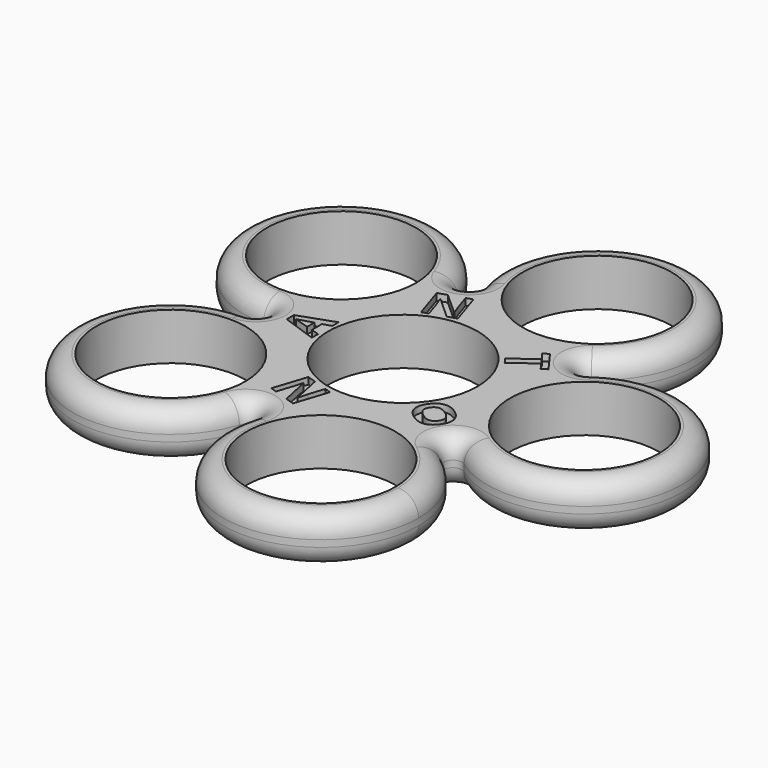
from build123d import *

# Parameters (mm, degrees)
F1_R         = 11.1
F2_DEPTH     = 3.5
F3_R         = 3
F4_TEXT_SIZE = 7.2184329232
F5_DEPTH     = 1


# Not quite as in the source:
# - Text() gives the source's letters only with a copy of the font that has no kerning and outlines rounded to 1/6400 em; it was checked with that copy


with BuildPart() as f2:
    # F1 (on Top) → F2 (new body, symmetric)
    with BuildSketch(Plane.XY):
        with BuildLine():
            ThreePointArc((18.4771138418, -11.7307464184), (33.5828622462, -12.9195946007), (41.5, 0))
            ThreePointArc((41.5, 0), (33.5828622462, 12.9195946007), (18.4771138418, 11.7307464184))
            ThreePointArc((18.4771138418, 11.7307464184), (12.5, 0), (18.4771138418, -11.7307464184))
        make_face()
        with Locations((27, 0)):
            Circle(F1_R, mode=Mode.SUBTRACT)
        with BuildLine():
            ThreePointArc((18.4771138418, -11.7307464184), (12.5, 0), (18.4771138418, 11.7307464184))
            ThreePointArc((18.4771138418, 11.7307464184), (16.5632128725, 12.0338785523), (16.8663450064, 13.9477795215))
            ThreePointArc((16.8663450064, 13.9477795215), (3.8627124297, 11.8882064537), (-5.4468606382, 21.1977795215))
            ThreePointArc((-5.4468606382, 21.1977795215), (-6.3265843544, 19.4712245141), (-8.0531393618, 20.3509482303))
            ThreePointArc((-8.0531393618, 20.3509482303), (-7.5219779095, 18.138501555), (-7.3434588481, 15.8702018119))
            ThreePointArc((-7.3434588481, 15.8702018119), (-11.5904105209, 5.6171534847), (-21.8434588481, 1.3702018119))
            ThreePointArc((-21.8434588481, 1.3702018119), (-20.4732570362, 0), (-21.8434588481, -1.3702018119))
            ThreePointArc((-21.8434588481, -1.3702018119), (-11.5904105209, -5.6171534847), (-7.3434588481, -15.8702018119))
            ThreePointArc((-7.3434588481, -15.8702018119), (-7.5219779095, -18.138501555), (-8.0531393618, -20.3509482303))
            ThreePointArc((-8.0531393618, -20.3509482303), (-6.3265843544, -19.4712245141), (-5.4468606382, -21.1977795215))
            ThreePointArc((-5.4468606382, -21.1977795215), (3.8627124297, -11.8882064537), (16.8663450064, -13.9477795215))
            ThreePointArc((16.8663450064, -13.9477795215), (16.5632128725, -12.0338785523), (18.4771138418, -11.7307464184))
        make_face()
        Circle(F1_R, mode=Mode.SUBTRACT)
        with BuildLine():
            ThreePointArc((-5.4468606382, 21.1977795215), (3.8627124297, 11.8882064537), (16.8663450064, 13.9477795215))
            ThreePointArc((16.8663450064, 13.9477795215), (21.2630534489, 19.0956636937), (22.8434588481, 25.67852594))
            ThreePointArc((22.8434588481, 25.67852594), (6.075159105, 40.0000068786), (-5.4468606382, 21.1977795215))
        make_face()
        with Locations((8.3434588481, 25.67852594)):
            Circle(F1_R, mode=Mode.SUBTRACT)
        with BuildLine():
            ThreePointArc((22.8434588481, -25.67852594), (21.2630534489, -19.0956636937), (16.8663450064, -13.9477795215))
            ThreePointArc((16.8663450064, -13.9477795215), (3.8627124297, -11.8882064537), (-5.4468606382, -21.1977795215))
            ThreePointArc((-5.4468606382, -21.1977795215), (6.075159105, -40.0000068786), (22.8434588481, -25.67852594))
        make_face()
        with Locations((8.3434588481, -25.67852594)):
            Circle(F1_R, mode=Mode.SUBTRACT)
        with BuildLine():
            ThreePointArc((-7.3434588481, 15.8702018119), (-7.5219779095, 18.138501555), (-8.0531393618, 20.3509482303))
            ThreePointArc((-8.0531393618, 20.3509482303), (-33.5742052666, 24.3930879701), (-21.8434588481, 1.3702018119))
            ThreePointArc((-21.8434588481, 1.3702018119), (-11.5904105209, 5.6171534847), (-7.3434588481, 15.8702018119))
        make_face()
        with Locations((-21.8434588481, 15.8702018119)):
            Circle(F1_R, mode=Mode.SUBTRACT)
        with BuildLine():
            ThreePointArc((-21.8434588481, -1.3702018119), (-33.5742052666, -24.3930879701), (-8.0531393618, -20.3509482303))
            ThreePointArc((-8.0531393618, -20.3509482303), (-7.5219779095, -18.138501555), (-7.3434588481, -15.8702018119))
            ThreePointArc((-7.3434588481, -15.8702018119), (-11.5904105209, -5.6171534847), (-21.8434588481, -1.3702018119))
        make_face()
        with Locations((-21.8434588481, -15.8702018119)):
            Circle(F1_R, mode=Mode.SUBTRACT)
    extrude(amount=F2_DEPTH, both=True)

    # F3
    f3_edges = [f2.edges().sort_by_distance(p)[0] for p in [
        (-33.574205, -24.393088, 3.5),
        (-33.574205, -24.393088, -3.5),
    ]]
    fillet(f3_edges, radius=F3_R)

    # F4 (on face) → F5 (cut, symmetric)
    with BuildSketch(Plane.XY.offset(3.5)):
        with Locations(Location((-11.5846967189, -2.4733702824), (0, 0, 90))):
            Text('A', F4_TEXT_SIZE, font='Open Sans', font_style=FontStyle.BOLD, text_align=(TextAlign.LEFT, TextAlign.BOTTOM))
        with Locations(Location((-6.3101283431, 10.2808768785), (0, 0, 18))):
            Text('N', F4_TEXT_SIZE, font='Open Sans', font_style=FontStyle.BOLD, text_align=(TextAlign.LEFT, TextAlign.BOTTOM))
        with Locations(Location((8.2989238401, 8.7424773108), (0, 0, -54))):
            Text('T', F4_TEXT_SIZE, font='Open Sans', font_style=FontStyle.BOLD, text_align=(TextAlign.LEFT, TextAlign.BOTTOM))
        with Locations(Location((11.122600367, -4.7498141065), (0, 0, -126))):
            Text('O', F4_TEXT_SIZE, font='Open Sans', font_style=FontStyle.BOLD, text_align=(TextAlign.LEFT, TextAlign.BOTTOM))
        with Locations(Location((-0.7597079111, -12.0412665495), (0, 0, 162))):
            Text('N', F4_TEXT_SIZE, font='Open Sans', font_style=FontStyle.BOLD, text_align=(TextAlign.LEFT, TextAlign.BOTTOM))
    extrude(amount=F5_DEPTH, both=True, mode=Mode.SUBTRACT)


solid = f2.part
